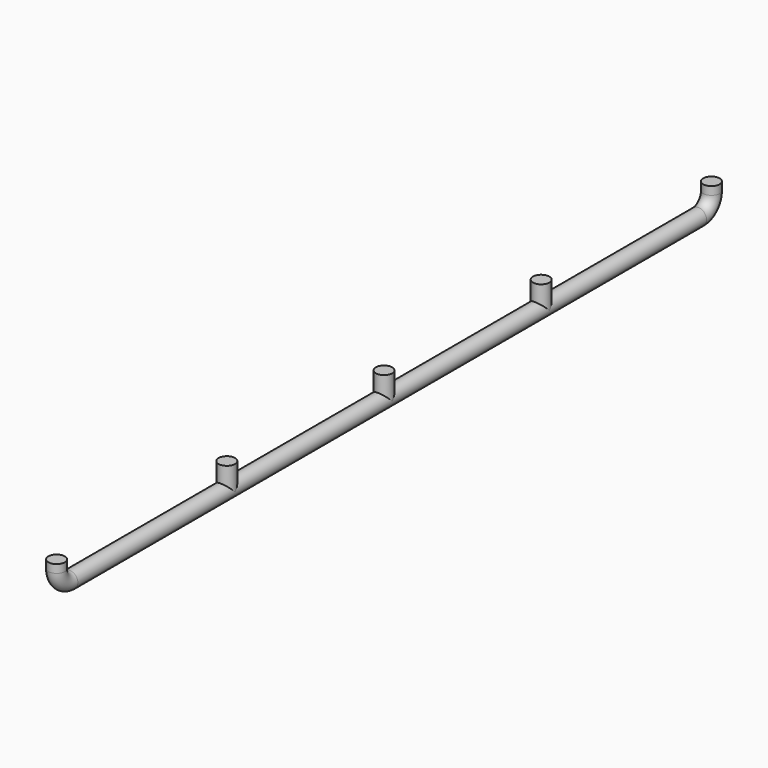
from build123d import *

# Parameters (mm, degrees)
F0_R          = 12.7
F1_DEPTH      = 609.6
F1_DEPTH_BACK = 609.6
F3_R          = 12.7
F8_R          = 12.7


# Not quite as in the source:
# - a pattern or mirror of a feature is missing from the dataset's text; its kind, count and spacing are read off the source's solid


with BuildPart() as f1:
    # F0 (on Front) → F1 (new body, two sides)
    with BuildSketch(Plane.XZ) as f1_sk:
        Circle(F0_R)
    extrude(amount=F1_DEPTH)
    extrude(f1_sk.sketch, amount=-F1_DEPTH_BACK)

    # F5: sweep along a path in F4
    with BuildLine(Plane.YZ) as f5_path:
        ThreePointArc((609.6, 0), (627.5605122421, 7.4394877579), (635, 25.4))
        Line((635, 25.4), (635, 38.1))
    # F3 (on offset) → F5 (sweep)
    with BuildSketch(Plane.XY.offset(38.1)):
        with Locations((0, 635)):
            Circle(F3_R)
    f5 = sweep(path=f5_path.line)

    # F5_copies: F5 across plane
    add(f5.mirror(Plane(origin=(0, 0, 0), x_dir=(0, 0, -1), z_dir=(0, -1, 0))))

    # F8 (on offset) → F9 (join, up to the next surface of F1)
    with BuildSketch(Plane.XY.offset(38.1)):
        with Locations((0, 304.8)):
            Circle(F8_R)
        with Locations((0, -304.8)):
            Circle(F8_R)
        Circle(F8_R)
    extrude(until=Until.NEXT, dir=(0, 0, -1))


solid = f1.part
